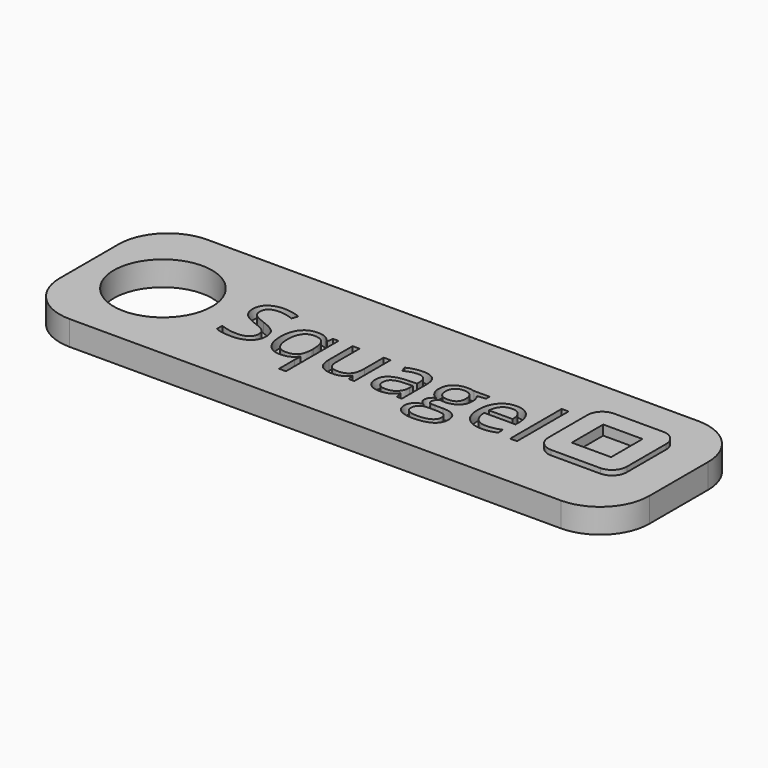
from build123d import *

# Parameters (mm, degrees)
F0_W         = 120
F0_H         = 35
F0_R         = 10
F1_DEPTH     = 5
F2_R         = 10
F3_TEXT_SIZE = 17.2697369837
F4_DEPTH     = 2
F5_W         = 16
F5_H         = 16
F5_W_2       = 8
F5_H_2       = 8
F6_DEPTH     = 1
F7_DEPTH     = 1
F8_R         = 3


# Not quite as in the source:
# - Text() gives the source's letters only with a copy of the font that has no kerning and outlines rounded to 1/6400 em; it was checked with that copy


with BuildPart() as f1:
    # F0 (on Top) → F1 (new body)
    with BuildSketch(Plane.XY):
        Rectangle(F0_W, F0_H)
        with Locations((-45, 0)):
            Circle(F0_R, mode=Mode.SUBTRACT)
    extrude(amount=F1_DEPTH)

    # F2
    f2_edges = [f1.edges().sort_by_distance(p)[0] for p in [
        (-60, -17.5, 2.5),
        (-60, 17.5, 2.5),
        (60, -17.5, 2.5),
        (60, 17.5, 2.5),
    ]]
    fillet(f2_edges, radius=F2_R)

    # F3 (on face) → F4 (cut)
    with BuildSketch(Plane.XY.offset(5)):
        with Locations((-30.4934233427, -5.9210527688)):
            Text('Squagel', F3_TEXT_SIZE, font='Open Sans', text_align=(TextAlign.LEFT, TextAlign.BOTTOM))
    extrude(amount=-F4_DEPTH, mode=Mode.SUBTRACT)

    # F5 (on face) → F6 (join)
    with BuildSketch(Plane.XY.offset(5)):
        with Locations((44.1184254289, 1.6381574217)):
            Rectangle(F5_W, F5_H)
        with Locations((44.1184254289, 1.6381574217)):
            Rectangle(F5_W_2, F5_H_2, mode=Mode.SUBTRACT)
    extrude(amount=F6_DEPTH)

    # F7 (cut): a face of the model
    f7_faces = [f1.faces().sort_by_distance(p)[0] for p in [
        (44.1184254289, 1.6381574217, 5),
    ]]
    extrude(f7_faces, amount=-F7_DEPTH, mode=Mode.SUBTRACT)

    # F8
    f8_edges = [f1.edges().sort_by_distance(p)[0] for p in [
        (52.118425, -6.361843, 5.5),
        (36.118425, -6.361843, 5.5),
        (36.118425, 9.638157, 5.5),
        (52.118425, 9.638157, 5.5),
    ]]
    fillet(f8_edges, radius=F8_R)


solid = f1.part
